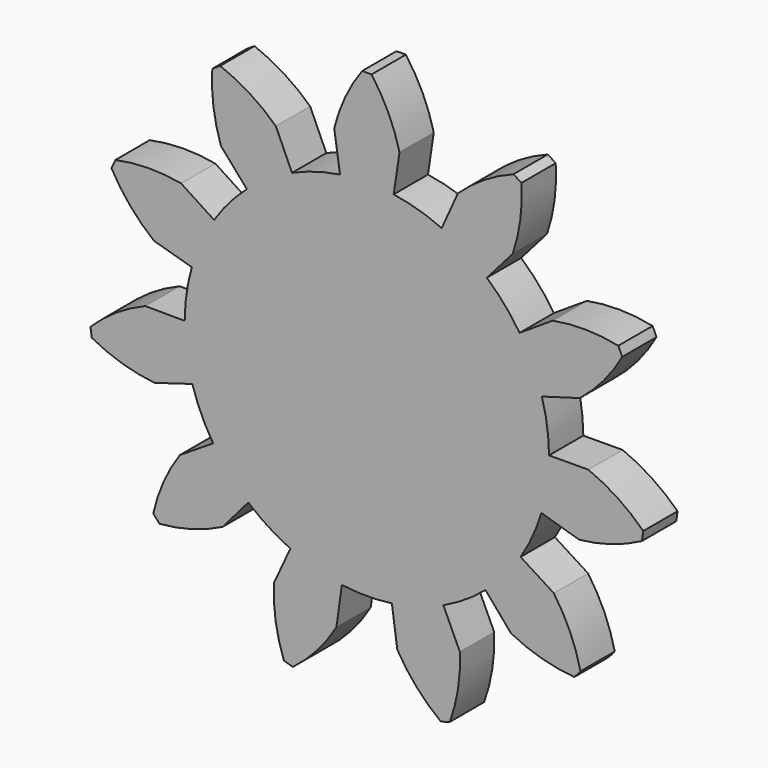
from build123d import *

# Parameters (mm, degrees)
F2_DEPTH        = 2.5
F2_COPIES_COUNT = 11
F3_DEPTH        = 2.5


# Not quite as in the source:
# - a pattern or mirror of a feature is missing from the dataset's text; its kind, count and spacing are read off the source's solid


with BuildPart() as f2:
    # F1 (on Front) → F2 (new body)
    with BuildSketch(Plane.XZ):
        with BuildLine():
            ThreePointArc((1.9034310201, 12.7798019983), (1.2593174989, 14.5936400637), (0.2749085502, 16.2476744579))
            ThreePointArc((0.2749085502, 16.2476744579), (0, 16.25), (-0.2749085502, 16.2476744579))
            ThreePointArc((-0.2749085502, 16.2476744579), (-1.2593174989, 14.5936400637), (-1.9034310201, 12.7798019983))
            Line((-1.9034310201, 12.7798019983), (-1.5652278506, 10.5090763998))
            ThreePointArc((-1.5652278506, 10.5090763998), (0, 10.625), (1.5652278506, 10.5090763998))
            Line((1.5652278506, 10.5090763998), (1.9034310201, 12.7798019983))
        make_face()
    extrude(amount=F2_DEPTH)


with BuildPart() as f2_copies_1:
    # F2_copies: instance of F2
    add(f2.part.rotate(Axis((0, 0, 0), (0, 1, 0)), 1 * 360 / F2_COPIES_COUNT))


with BuildPart() as f2_copies_2:
    # F2_copies: instance of F2
    add(f2.part.rotate(Axis((0, 0, 0), (0, 1, 0)), 2 * 360 / F2_COPIES_COUNT))


with BuildPart() as f2_copies_3:
    # F2_copies: instance of F2
    add(f2.part.rotate(Axis((0, 0, 0), (0, 1, 0)), 3 * 360 / F2_COPIES_COUNT))


with BuildPart() as f2_copies_4:
    # F2_copies: instance of F2
    add(f2.part.rotate(Axis((0, 0, 0), (0, 1, 0)), 4 * 360 / F2_COPIES_COUNT))


with BuildPart() as f2_copies_5:
    # F2_copies: instance of F2
    add(f2.part.rotate(Axis((0, 0, 0), (0, 1, 0)), 5 * 360 / F2_COPIES_COUNT))


with BuildPart() as f2_copies_6:
    # F2_copies: instance of F2
    add(f2.part.rotate(Axis((0, 0, 0), (0, 1, 0)), 6 * 360 / F2_COPIES_COUNT))


with BuildPart() as f2_copies_7:
    # F2_copies: instance of F2
    add(f2.part.rotate(Axis((0, 0, 0), (0, 1, 0)), 7 * 360 / F2_COPIES_COUNT))


with BuildPart() as f2_copies_8:
    # F2_copies: instance of F2
    add(f2.part.rotate(Axis((0, 0, 0), (0, 1, 0)), 8 * 360 / F2_COPIES_COUNT))


with BuildPart() as f2_copies_9:
    # F2_copies: instance of F2
    add(f2.part.rotate(Axis((0, 0, 0), (0, 1, 0)), 9 * 360 / F2_COPIES_COUNT))


with BuildPart() as f2_copies_10:
    # F2_copies: instance of F2
    add(f2.part.rotate(Axis((0, 0, 0), (0, 1, 0)), 10 * 360 / F2_COPIES_COUNT))


with BuildPart() as f2_1:
    add(f2.part)

    add(f2_copies_1.part)  # F3 merges F2_copies_1

    add(f2_copies_2.part)  # F3 merges F2_copies_2

    add(f2_copies_3.part)  # F3 merges F2_copies_3

    add(f2_copies_4.part)  # F3 merges F2_copies_4

    add(f2_copies_5.part)  # F3 merges F2_copies_5

    add(f2_copies_6.part)  # F3 merges F2_copies_6

    add(f2_copies_7.part)  # F3 merges F2_copies_7

    add(f2_copies_8.part)  # F3 merges F2_copies_8

    add(f2_copies_9.part)  # F3 merges F2_copies_9

    add(f2_copies_10.part)  # F3 merges F2_copies_10
    # F1 (on Front) → F3 (join)
    with BuildSketch(Plane.XZ):
        with BuildLine():
            ThreePointArc((10.625, 0), (8.0473961911, 6.9375816784), (1.5652278506, 10.5090763998))
            ThreePointArc((1.5652278506, 10.5090763998), (0, 10.625), (-1.5652278506, 10.5090763998))
            ThreePointArc((-1.5652278506, 10.5090763998), (-6.9375816784, -8.0473961911), (10.625, 0))
        make_face()
    extrude(amount=F3_DEPTH)


solid = f2_1.part
